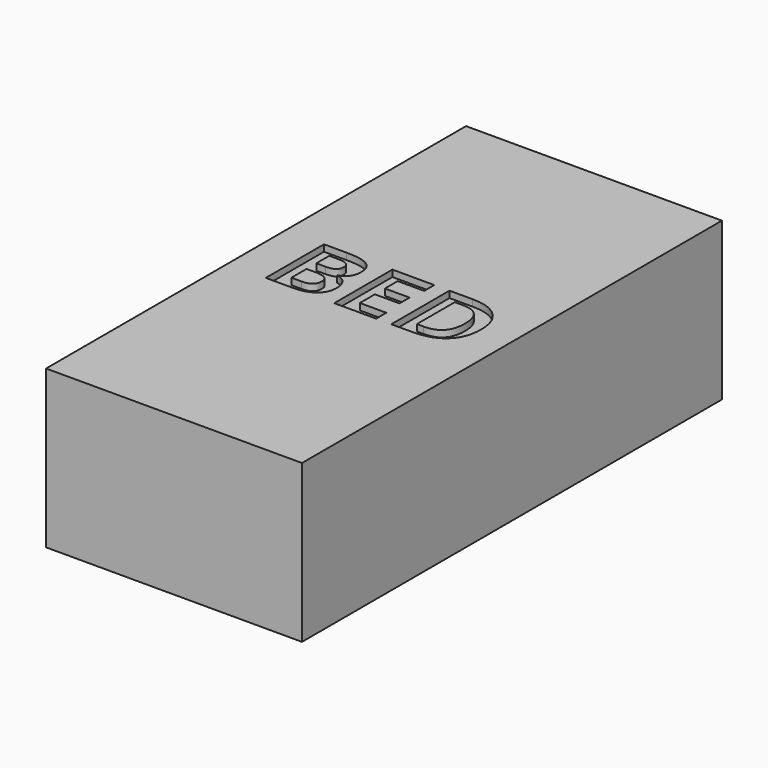
from build123d import *

# Parameters (mm, degrees)
F0_W         = 990.6
F0_H         = 2032
F1_DEPTH     = 609.6
F2_TEXT_SIZE = 394.3380382326
F3_DEPTH     = 25.4


# Not quite as in the source:
# - Text() gives the source's letters only with a copy of the font that has no kerning and outlines rounded to 1/6400 em; it was checked with that copy


with BuildPart() as f1:
    # F0 (on Top) → F1 (new body)
    with BuildSketch(Plane.XY):
        with Locations((495.3, 1016)):
            Rectangle(F0_W, F0_H)
    extrude(amount=F1_DEPTH)

    # F2 (on face) → F3 (cut)
    with BuildSketch(Plane.XY.offset(609.6)):
        with Locations((112.5946342945, 878.0448436737)):
            Text('BED', F2_TEXT_SIZE, font='Open Sans', font_style=FontStyle.BOLD, text_align=(TextAlign.LEFT, TextAlign.BOTTOM))
    extrude(amount=-F3_DEPTH, mode=Mode.SUBTRACT)


solid = f1.part
